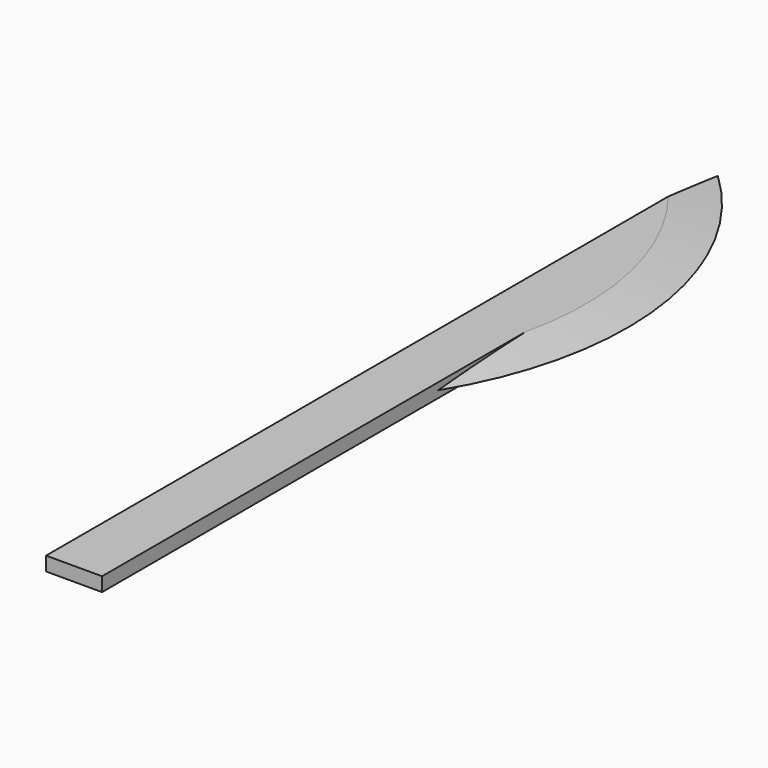
from build123d import *

# Parameters (mm, degrees)
F1_DEPTH = 1.27
F2_SIZE2 = 0.635
F2_SIZE  = 3.81
F3_SIZE2 = 3.80999
F3_SIZE  = 0.63499


# Not quite as in the source:
# - a fillet or chamfer is up to 0.001 mm smaller than in the source, because OpenCascade refuses the exact size


with BuildPart() as f1:
    # F0 (on Top) → F1 (new body)
    with BuildSketch(Plane.XY):
        with BuildLine():
            Line((-36.8330654015, 25.4), (-36.8330654015, 0))
            Line((-36.8330654015, 0), (-31.7530654015, 0))
            Line((-31.7530654015, 0), (-31.7530654015, 25.4))
            Line((-31.7530654015, 25.4), (-31.7530654015, 38.1))
            ThreePointArc((-31.7530654015, 38.1), (-27.5303919686, 58.0516897911), (-36.8330654015, 76.2))
            Line((-36.8330654015, 76.2), (-36.8330654015, 25.4))
        make_face()
    extrude(amount=F1_DEPTH)

    # F2
    f2_edges = [f1.edges().sort_by_distance(p)[0] for p in [
        (-27.530392, 58.05169, 1.27),
    ]]
    f2_side = f1.faces().sort_by_distance((-33.424726, 40.272923, 1.27))[0]
    chamfer(f2_edges, length=F2_SIZE, length2=F2_SIZE2, reference=f2_side)

    # F3 (size 0.635 and 3.81 in the source; OpenCascade refuses exactly that, so slightly less here)
    f3_edges = [f1.edges().sort_by_distance(p)[0] for p in [
        (-27.530392, 58.05169, 0),
    ]]
    f3_side = f1.faces().sort_by_distance((-27.530392, 58.05169, 0.3175))[0]
    chamfer(f3_edges, length=F3_SIZE, length2=F3_SIZE2, reference=f3_side)


solid = f1.part
